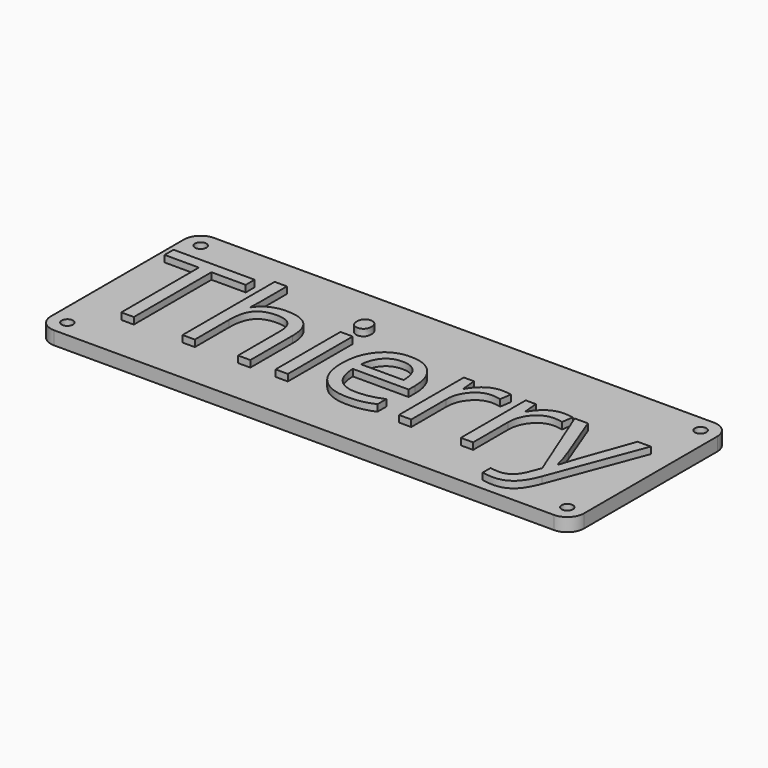
from build123d import *

# Parameters (mm, degrees)
F0_W         = 160
F0_H         = 60
F1_DEPTH     = 4
F2_R         = 5
F4_D         = 3.4
F5_TEXT_SIZE = 45.4761010284
F6_DEPTH     = 2


# Not quite as in the source:
# - Text() gives the source's letters only with a copy of the font that has no kerning and outlines rounded to 1/6400 em; it was checked with that copy


with BuildPart() as f1:
    # F0 (on Top) → F1 (new body)
    with BuildSketch(Plane.XY):
        Rectangle(F0_W, F0_H)
    extrude(amount=F1_DEPTH)

    # F2
    f2_edges = [f1.edges().sort_by_distance(p)[0] for p in [
        (80, -30, 2),
        (80, 30, 2),
        (-80, -30, 2),
        (-80, 30, 2),
    ]]
    fillet(f2_edges, radius=F2_R)

    # F4 (through all)
    with Locations(Plane.XY.offset(4)):
        with Locations((75, 25), (75, -25), (-75, -25), (-75, 25)):
            Hole(F4_D / 2)

    # F5 (on face) → F6 (join)
    with BuildSketch(Plane.XY.offset(4)):
        with Locations((-76.6587853432, -16.0726485774)):
            Text('Thierry', F5_TEXT_SIZE, font='Open Sans', text_align=(TextAlign.LEFT, TextAlign.BOTTOM))
    extrude(amount=F6_DEPTH)


solid = f1.part
